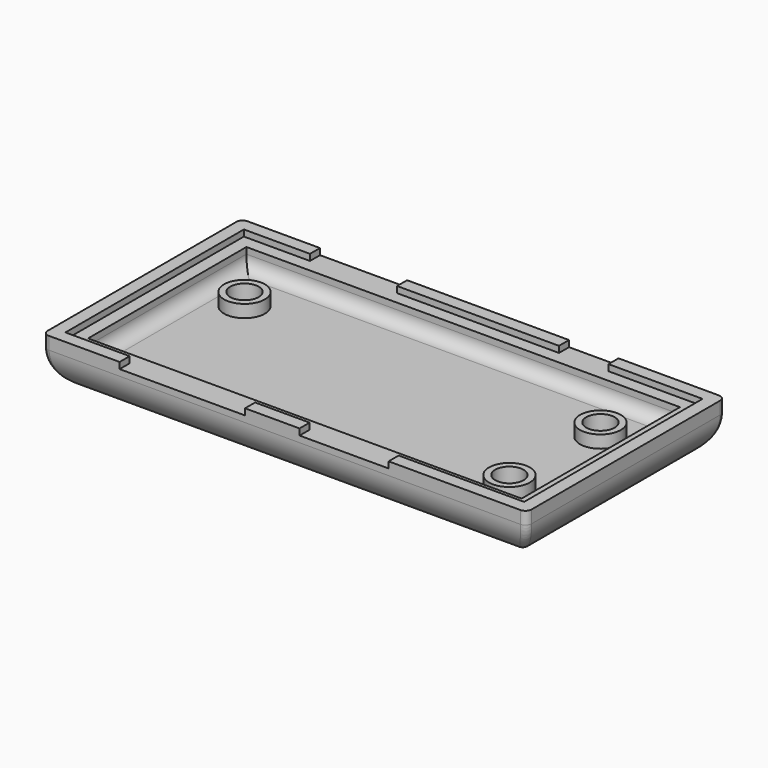
from build123d import *

# Parameters (mm, degrees)
F0_W      = 82.55
F0_H      = 34.925
F0_R      = 2.8702
F1_DEPTH  = 5.08
F4_R      = 1.27
F5_W      = 17.59966
F5_H      = 1.27
F5_W_2    = 9.99998
F6_DEPTH  = 3.556
F7_R      = 4.1275
F7_R_2    = 2.8702
F8_DEPTH  = 2.54
F9_W      = 18.00098
F9_H      = 1.27
F9_W_2    = 25.3492
F10_DEPTH = 5.08


with BuildPart() as f1:
    # F0 (on Top) → F1 (new body)
    with BuildSketch(Plane.XY):
        Rectangle(F0_W, F0_H)
        with Locations((35.75, -13)):
            Circle(F0_R, mode=Mode.SUBTRACT)
        with Locations((-36, 9.75)):
            Circle(F0_R, mode=Mode.SUBTRACT)
        with Locations((35.75, 10)):
            Circle(F0_R, mode=Mode.SUBTRACT)
    extrude(amount=F1_DEPTH)

    # F3: sweep along a path in F3_path
    with BuildLine(Plane(origin=(-41.275, 17.4625, 5.08), x_dir=(0, -1, 0), z_dir=(0, 0, -1))) as f3_path:
        Line((0, 0), (34.925, 0))
        Line((34.925, 0), (34.925, -82.55))
        Line((34.925, -82.55), (0, -82.55))
        Line((0, -82.55), (0, 0))
    # F2 (on Front) → F3 (sweep)
    with BuildSketch(Plane.XZ):
        with BuildLine():
            Line((-41.275, 0), (-41.275, 5.08))
            ThreePointArc((-41.275, 5.08), (-43.0710512242, 5.8239487758), (-43.815, 7.62))
            Line((-43.815, 7.62), (-43.815, 8.89))
            Line((-43.815, 8.89), (-46.355, 8.89))
            Line((-46.355, 8.89), (-46.355, 10.16))
            Line((-46.355, 10.16), (-48.895, 10.16))
            Line((-48.895, 10.16), (-48.895, 7.62))
            ThreePointArc((-48.895, 7.62), (-46.6631536726, 2.2318463274), (-41.275, 0))
        make_face()
    sweep(path=f3_path.line, transition=Transition.RIGHT)

    # F4
    f4_edges = [f1.edges().sort_by_distance(p)[0] for p in [
        (46.663154, 22.850654, 2.231846),
        (-46.663154, 22.850654, 2.231846),
        (-46.663154, -22.850654, 2.231846),
        (46.663154, -22.850654, 2.231846),
        (48.895, 25.0825, 8.89),
        (-48.895, 25.0825, 8.89),
        (-48.895, -25.0825, 8.89),
        (48.895, -25.0825, 8.89),
    ]]
    fillet(f4_edges, radius=F4_R)

    # F5 (on face) → F6 (cut)
    with BuildSketch(Plane(origin=(0, 25.0825, 0), x_dir=(-1, 0, 0), z_dir=(0, 1, 0))):
        with Locations((24.20069, 9.525)):
            Rectangle(F5_W, F5_H)
        with Locations((-22.33125, 9.525)):
            Rectangle(F5_W_2, F5_H)
    extrude(amount=-F6_DEPTH, mode=Mode.SUBTRACT)

    # F7 (on face) → F8 (join)
    with BuildSketch(Plane.XY.offset(5.08)):
        with Locations((-36, 9.75)):
            Circle(F7_R)
        with Locations((-36, 9.75)):
            Circle(F7_R_2, mode=Mode.SUBTRACT)
        with Locations((35.75, 10)):
            Circle(F7_R)
        with Locations((35.75, 10)):
            Circle(F7_R_2, mode=Mode.SUBTRACT)
        with Locations((35.75, -13)):
            Circle(F7_R)
        with Locations((35.75, -13)):
            Circle(F7_R_2, mode=Mode.SUBTRACT)
    extrude(amount=F8_DEPTH)

    # F9 (on face) → F10 (cut)
    with BuildSketch(Plane.XZ.offset(25.0825)):
        with Locations((11.99853, 9.525)):
            Rectangle(F9_W, F9_H)
        with Locations((-20.69422, 9.525)):
            Rectangle(F9_W_2, F9_H)
    extrude(amount=-F10_DEPTH, mode=Mode.SUBTRACT)


solid = f1.part
